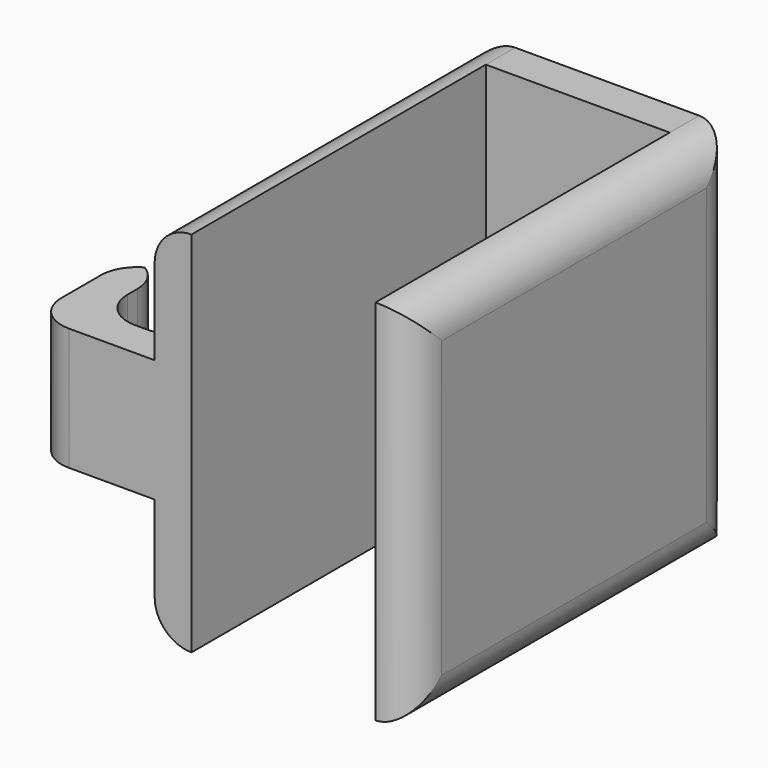
from build123d import *

# Parameters (mm, degrees)
F1_DEPTH    = 30
F2_START    = 10
F2_DEPTH    = 10
F3_T1_DEPTH = 10
F3_T3_DEPTH = 25
F3_T5_DEPTH = 48
F3_T7_DEPTH = 45


# Not quite as in the source:
# - a fillet or chamfer that OpenCascade refuses, or shapes differently, is made with other operations: its cross-section is extruded or revolved along the edge and cut away or added


with BuildPart() as f1:
    # F0 (on Top) → F1 (new body)
    with BuildSketch(Plane.XY):
        Polygon((7.5, 30), (7.5, 0), (10.5, 0), (10.5, 33), (-10.5, 33), (-10.5, 3), (-10.5, 0), (-7.5, 0), (-7.5, 30), align=None)
    extrude(amount=F1_DEPTH)

    # F0 (on Top) → F2 (join)
    with BuildSketch(Plane.XY.offset(F2_START)):
        Polygon((7.5, 30), (7.5, 0), (10.5, 0), (10.5, 33), (-10.5, 33), (-10.5, 3), (-10.5, 0), (-7.5, 0), (-7.5, 30), align=None)
        Polygon((-10.5, 0), (-10.5, 3), (-17.5, 3), (-17.5, 10), (-20.5, 10), (-20.5, 0), align=None)
    extrude(amount=F2_DEPTH)

    # F3: fillet of radius 3 on 12 edges, made by hand

    # F3_s2 → F3_t1 (join)
    with BuildSketch(Plane.XY.offset(10)):
        with BuildLine():
            ThreePointArc((-10.5, 6), (-11.3786796564, 3.8786796564), (-13.5, 3))
            Line((-13.5, 3), (-10.5, 3))
            Line((-10.5, 3), (-10.5, 6))
        make_face()
        with BuildLine():
            ThreePointArc((-17.5, 6), (-16.6213203436, 3.8786796564), (-14.5, 3))
            Line((-14.5, 3), (-17.5, 3))
            Line((-17.5, 3), (-17.5, 6))
        make_face()
    extrude(amount=F3_T1_DEPTH)

    # F3_s4 → F3_t3 (cut)
    with BuildSketch(Plane.XY.offset(2.5)):
        with BuildLine():
            ThreePointArc((-20.5, 10), (-18.3786796564, 9.1213203436), (-17.5, 7))
            Line((-17.5, 7), (-17.5, 10))
            Line((-17.5, 10), (-20.5, 10))
        make_face()
        with BuildLine():
            ThreePointArc((-20.5, 3), (-19.6213203436, 0.8786796564), (-17.5, 0))
            Line((-17.5, 0), (-20.5, 0))
            Line((-20.5, 0), (-20.5, 3))
        make_face()
        with BuildLine():
            ThreePointArc((-20.5, 7), (-19.6213203436, 9.1213203436), (-17.5, 10))
            Line((-17.5, 10), (-20.5, 10))
            Line((-20.5, 10), (-20.5, 7))
        make_face()
    extrude(amount=F3_T3_DEPTH, mode=Mode.SUBTRACT)

    # F3_s6 → F3_t5 (cut)
    with BuildSketch(Plane.XZ.offset(-40.5)):
        with BuildLine():
            ThreePointArc((-10.5, 27), (-9.6213203436, 29.1213203436), (-7.5, 30))
            Line((-7.5, 30), (-10.5, 30))
            Line((-10.5, 30), (-10.5, 27))
        make_face()
        with BuildLine():
            ThreePointArc((10.5, 3), (9.6213203436, 0.8786796564), (7.5, 0))
            Line((7.5, 0), (10.5, 0))
            Line((10.5, 0), (10.5, 3))
        make_face()
        with BuildLine():
            ThreePointArc((10.5, 27), (9.6213203436, 29.1213203436), (7.5, 30))
            Line((7.5, 30), (10.5, 30))
            Line((10.5, 30), (10.5, 27))
        make_face()
        with BuildLine():
            ThreePointArc((-10.5, 3), (-9.6213203436, 0.8786796564), (-7.5, 0))
            Line((-7.5, 0), (-10.5, 0))
            Line((-10.5, 0), (-10.5, 3))
        make_face()
    extrude(amount=F3_T5_DEPTH, mode=Mode.SUBTRACT)

    # F3_s8 → F3_t7 (cut)
    with BuildSketch(Plane.XY.offset(-7.5)):
        with BuildLine():
            ThreePointArc((7.5, 0), (9.6213203436, 0.8786796564), (10.5, 3))
            Line((10.5, 3), (10.5, 0))
            Line((10.5, 0), (7.5, 0))
        make_face()
        with BuildLine():
            ThreePointArc((10.5, 30), (9.6213203436, 32.1213203436), (7.5, 33))
            Line((7.5, 33), (10.5, 33))
            Line((10.5, 33), (10.5, 30))
        make_face()
        with BuildLine():
            ThreePointArc((-7.5, 33), (-9.6213203436, 32.1213203436), (-10.5, 30))
            Line((-10.5, 30), (-10.5, 33))
            Line((-10.5, 33), (-7.5, 33))
        make_face()
    extrude(amount=F3_T7_DEPTH, mode=Mode.SUBTRACT)


solid = f1.part
